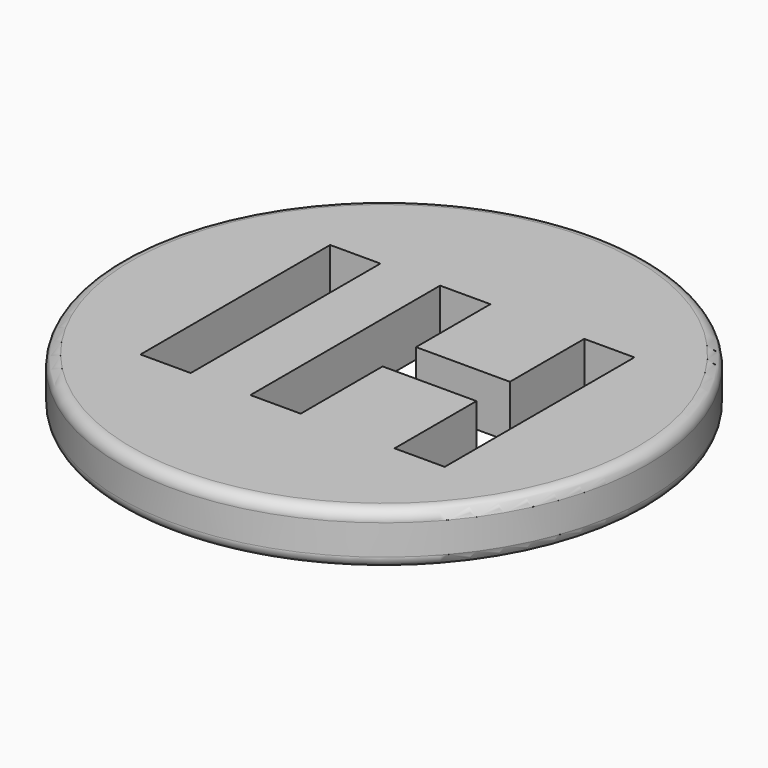
from build123d import *

# Parameters (mm, degrees)
F0_R         = 11.625
F1_DEPTH     = 2.33
F2_TEXT_SIZE = 14.6275062838
F3_DEPTH     = 2.331
F4_R         = 0.5


# Not quite as in the source:
# - Text() gives the source's letters only with a copy of the font that has no kerning and outlines rounded to 1/6400 em; it was checked with that copy


with BuildPart() as f1:
    # F0 (on Top) → F1 (new body)
    with BuildSketch(Plane.XY):
        Circle(F0_R)
    extrude(amount=F1_DEPTH)

    # F2 (on face) → F3 (cut, through all)
    with BuildSketch(Plane.XY.offset(2.33)):
        with Locations((-7.8314297315, -5.2659022622)):
            Text('IH', F2_TEXT_SIZE, font='Open Sans', font_style=FontStyle.BOLD, text_align=(TextAlign.LEFT, TextAlign.BOTTOM))
    extrude(amount=-F3_DEPTH, mode=Mode.SUBTRACT)

    # F4
    f4_edges = [f1.edges().sort_by_distance(p)[0] for p in [
        (-11.625, 0, 2.33),
        (-11.625, 0, 0),
    ]]
    fillet(f4_edges, radius=F4_R)


solid = f1.part
